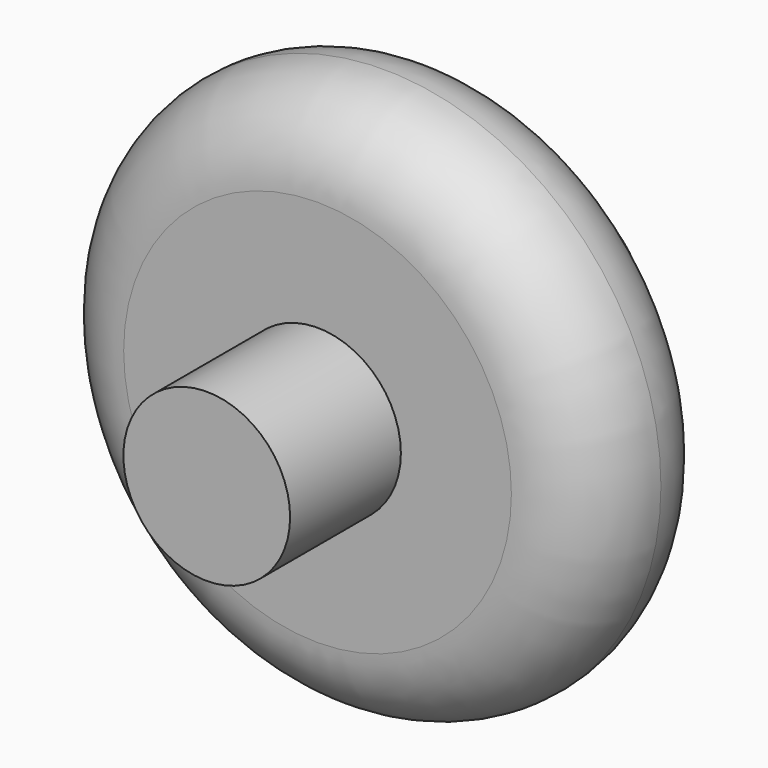
from build123d import *

# Parameters (mm, degrees)
F0_R     = 15.046961384
F1_DEPTH = 40
F0_R_2   = 50
F2_DEPTH = 15
F3_R     = 14.99999


# Not quite as in the source:
# - a fillet or chamfer is up to 0.001 mm smaller than in the source, because OpenCascade refuses the exact size


with BuildPart() as f1:
    # F0 (on Front) → F1 (new body, symmetric)
    with BuildSketch(Plane.XZ):
        Circle(F0_R)
    extrude(amount=F1_DEPTH, both=True)

    # F0 (on Front) → F2 (join, symmetric)
    with BuildSketch(Plane.XZ):
        Circle(F0_R_2)
        Circle(F0_R, mode=Mode.SUBTRACT)
    extrude(amount=F2_DEPTH, both=True)

    # F3 (radius 15 in the source; OpenCascade refuses exactly that, so slightly less here)
    f3_edges = [f1.edges().sort_by_distance(p)[0] for p in [
        (-50, -15, 0),
        (-50, 15, 0),
    ]]
    fillet(f3_edges, radius=F3_R)


solid = f1.part
